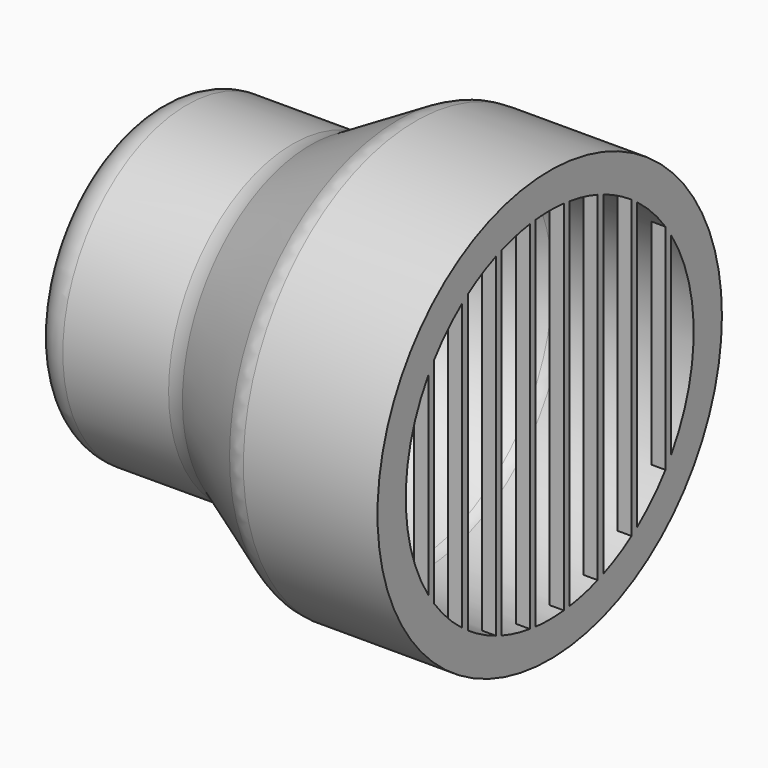
from build123d import *

# Parameters (mm, degrees)
F2_R     = 30.5
F3_DEPTH = 2
F5_DEPTH = 2
F6_R     = 4.99999
F7_R     = 3


# Not quite as in the source:
# - a fillet or chamfer is up to 0.001 mm smaller than in the source, because OpenCascade refuses the exact size
# - a feature names something its author has since deleted; it is built from what else it names


with BuildPart() as f1:
    # F0 (on Top) → F1 (revolve)
    with BuildSketch(Plane.XY):
        Polygon((-22.6666666667, 22), (-22.6666666667, 17), (0, 17), (14.7224318643, 25.5), (31.7224318643, 25.5), (31.7224318643, 30.5), (13.3826859022, 30.5), (-1.3397459622, 22), align=None)
    revolve(axis=Axis((-8.7595172226, 0, 0), (1, 0, 0)))

    # F2 (on face) → F3 (join)
    with BuildSketch(Plane.YZ.offset(31.7224318643)):
        Circle(F2_R)
    extrude(amount=F3_DEPTH)

    # F4 (on face) → F5 (cut, through all)
    with BuildSketch(Plane.YZ.offset(33.7224318643)):
        with BuildLine():
            ThreePointArc((20.5, 15.1657508881), (18.1785168447, 17.8827158264), (15.5, 20.2484567313))
            Line((15.5, 20.2484567313), (15.5, -20.2484567313))
            ThreePointArc((15.5, -20.2484567313), (18.1785168447, -17.8827158264), (20.5, -15.1657508881))
            Line((20.5, -15.1657508881), (20.5, 15.1657508881))
        make_face()
        with BuildLine():
            ThreePointArc((14.5, 20.9761769634), (12.0750373532, 22.4598190758), (9.5, 23.6643191324))
            Line((9.5, 23.6643191324), (9.5, -23.6643191324))
            ThreePointArc((9.5, -23.6643191324), (12.0750373532, -22.4598190758), (14.5, -20.9761769634))
            Line((14.5, -20.9761769634), (14.5, 20.9761769634))
        make_face()
        with BuildLine():
            ThreePointArc((8.5, 24.0416305603), (6.0307786652, 24.7765959868), (3.5, 25.2586618806))
            Line((3.5, 25.2586618806), (3.5, -25.2586618806))
            ThreePointArc((3.5, -25.2586618806), (6.0307786652, -24.7765959868), (8.5, -24.0416305603))
            Line((8.5, -24.0416305603), (8.5, 24.0416305603))
        make_face()
        with BuildLine():
            ThreePointArc((2.5, 25.3771550809), (1.2515081776, 25.4692702542), (0, 25.5))
            ThreePointArc((0, 25.5), (-1.2515081776, 25.4692702542), (-2.5, 25.3771550809))
            Line((-2.5, 25.3771550809), (-2.5, -25.3771550809))
            ThreePointArc((-2.5, -25.3771550809), (-1.2515081776, -25.4692702542), (0, -25.5))
            ThreePointArc((0, -25.5), (1.2515081776, -25.4692702542), (2.5, -25.3771550809))
            Line((2.5, -25.3771550809), (2.5, 25.3771550809))
        make_face()
        with BuildLine():
            Line((-3.5, -25.2586618806), (-3.5, 25.2586618806))
            ThreePointArc((-3.5, 25.2586618806), (-6.0307786652, 24.7765959868), (-8.5, 24.0416305603))
            Line((-8.5, 24.0416305603), (-8.5, -24.0416305603))
            ThreePointArc((-8.5, -24.0416305603), (-6.0307786652, -24.7765959868), (-3.5, -25.2586618806))
        make_face()
        with BuildLine():
            Line((-9.5, -23.6643191324), (-9.5, 23.6643191324))
            ThreePointArc((-9.5, 23.6643191324), (-12.0750373532, 22.4598190758), (-14.5, 20.9761769634))
            Line((-14.5, 20.9761769634), (-14.5, -20.9761769634))
            ThreePointArc((-14.5, -20.9761769634), (-12.0750373532, -22.4598190758), (-9.5, -23.6643191324))
        make_face()
        with BuildLine():
            Line((-15.5, -20.2484567313), (-15.5, 20.2484567313))
            ThreePointArc((-15.5, 20.2484567313), (-18.1785168447, 17.8827158264), (-20.5, 15.1657508881))
            Line((-20.5, 15.1657508881), (-20.5, -15.1657508881))
            ThreePointArc((-20.5, -15.1657508881), (-18.1785168447, -17.8827158264), (-15.5, -20.2484567313))
        make_face()
        with BuildLine():
            Line((-21.5, -13.7113092008), (-21.5, 13.7113092008))
            ThreePointArc((-21.5, 13.7113092008), (-25.5, 0), (-21.5, -13.7113092008))
        make_face()
        with BuildLine():
            ThreePointArc((25.5, 0), (24.4795833298, 7.1414284285), (21.5, 13.7113092008))
            Line((21.5, 13.7113092008), (21.5, -13.7113092008))
            ThreePointArc((21.5, -13.7113092008), (24.4795833298, -7.1414284285), (25.5, 0))
        make_face()
    extrude(amount=-F5_DEPTH, mode=Mode.SUBTRACT)

    # F6 (radius 5 in the source; OpenCascade refuses exactly that, so slightly less here)
    f6_edges = [f1.edges().sort_by_distance(p)[0] for p in [
        (-22.666667, -22, 0),
        (-1.339746, -22, 0),
        (13.382686, -30.5, 0),
    ]]
    fillet(f6_edges, radius=F6_R)

    # F7
    f7_edges = [f1.edges().sort_by_distance(p)[0] for p in [
        (14.722432, -25.5, 0),
        (0, -17, 0),
    ]]
    fillet(f7_edges, radius=F7_R)


solid = f1.part
